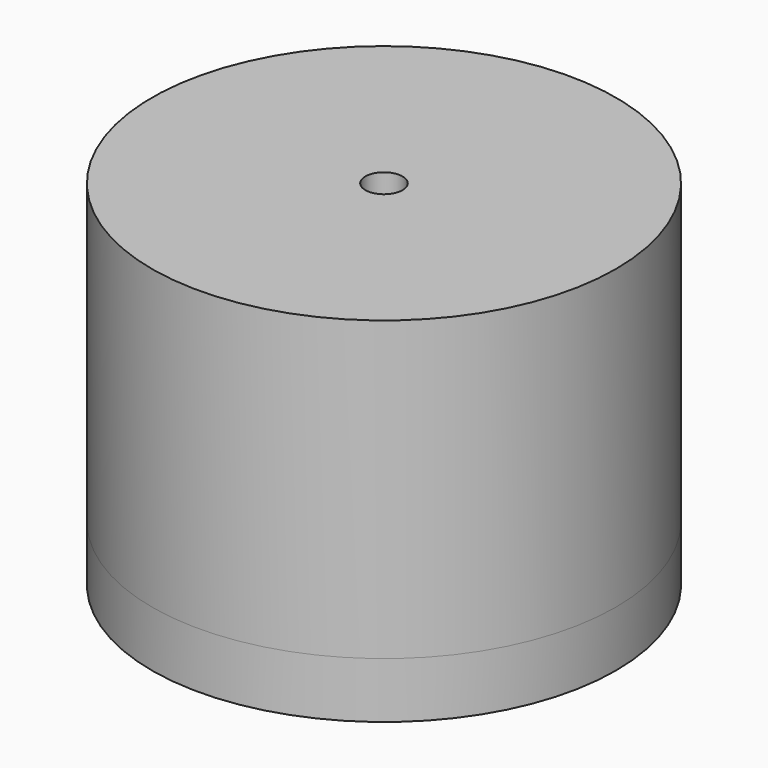
from build123d import *

# Parameters (mm, degrees)
F0_R     = 39.5915357934
F1_DEPTH = 9.525
F2_DEPTH = 50.8
F4_D     = 6.35
F4_2_D   = 6.35


# Not quite as in the source:
# - a feature names something its author has since deleted; it is built from what else it names


with BuildPart() as f1:
    # F0 (on Top) → F1 (new body, symmetric)
    with BuildSketch(Plane.XY):
        Circle(F0_R)
    extrude(amount=F1_DEPTH, both=True)

    # F4 (through all)
    with Locations(Plane.XY.offset(50.8)):
        with Locations((0, 0)):
            Hole(F4_D / 2)


with BuildPart() as f2:
    # F0 (on Top) → F2 (new body)
    with BuildSketch(Plane.XY):
        Circle(F0_R)
    extrude(amount=F2_DEPTH)

    # F4#2 (through all)
    with Locations(Plane.XY.offset(50.8)):
        with Locations((0, 0)):
            Hole(F4_2_D / 2)


solid = Compound([f1.part, f2.part])
